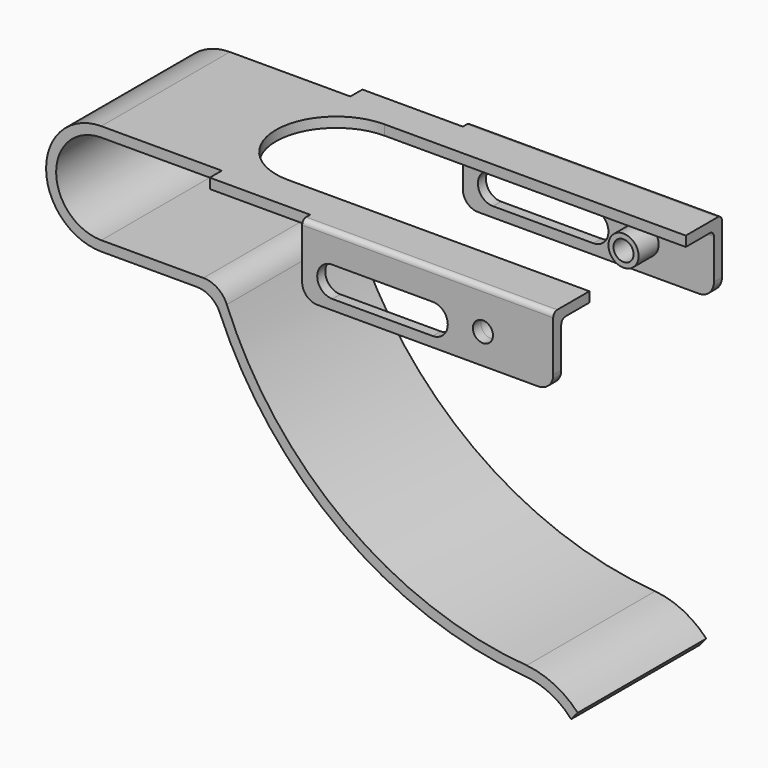
from build123d import *

# Parameters (mm, degrees)
F1_DEPTH  = 16
F2_W      = 70
F2_H      = 3
F3_DEPTH  = 2
F4_W      = 50
F4_H      = 14
F5_DEPTH  = 2
F6_R      = 1
F9_DEPTH  = 2
F11_DEPTH = 42.001
F13_D     = 4
F14_R     = 3
F14_R_2   = 2
F15_DEPTH = 5
F16_R     = 3


# Not quite as in the source:
# - a pattern or mirror of a feature is missing from the dataset's text; its kind, count and spacing are read off the source's solid


with BuildPart() as f1:
    # F0 (on Front) → F1 (new body)
    with BuildSketch(Plane.XZ):
        with BuildLine():
            ThreePointArc((0, -9), (-9, 0), (0, 9))
            Line((0, 9), (94, 9))
            Line((94, 9), (94, 11))
            Line((94, 11), (0, 11))
            ThreePointArc((0, 11), (-11, 0), (0, -11))
            Line((0, -11), (19, -11))
            ThreePointArc((19, -11), (21.7681124643, -11.8361612201), (23.6103896104, -14.064978646))
            ThreePointArc((23.6103896104, -14.064978646), (47.704208574, -44.4678662727), (84.0759449666, -57.9565459739))
            ThreePointArc((84.0759449666, -57.9565459739), (89.2804195373, -59.3196982134), (93.5865207758, -62.5449473062))
            Line((93.5865207758, -62.5449473062), (94.8828854905, -61))
            ThreePointArc((94.8828854905, -61), (90.2510294077, -57.5678191663), (84.7034264019, -56))
            ThreePointArc((84.7034264019, -56), (48.5673164119, -42.6217020739), (24.9861322889, -12.1467114099))
            ThreePointArc((24.9861322889, -12.1467114099), (23.1470623984, -9.8607704249), (20.3422845953, -9))
            Line((20.3422845953, -9), (0, -9))
        make_face()
    extrude(amount=F1_DEPTH)

    # F2 (on face) → F3 (join)
    with BuildSketch(Plane.XY.offset(11)):
        with Locations((59, -17.5)):
            Rectangle(F2_W, F2_H)
    extrude(amount=-F3_DEPTH)

    # F4 (on face) → F5 (join)
    with BuildSketch(Plane.XZ.offset(19)):
        with Locations((69, 4)):
            Rectangle(F4_W, F4_H)
    extrude(amount=F5_DEPTH)

    # F6
    f6_edges = [f1.edges().sort_by_distance(p)[0] for p in [
        (69, -21, 11),
        (69, -19, 9),
    ]]
    fillet(f6_edges, radius=F6_R)

    # F7: F1 across plane


with BuildPart() as f1_1:
    add(f1.part)
    add(f1.part.mirror(Plane.XZ))

    # F8 (on face) → F9 (cut)
    with BuildSketch(Plane.XY.offset(11)):
        with BuildLine():
            Line((94, 12), (34, 12))
            ThreePointArc((34, 12), (22, 0), (34, -12))
            Line((34, -12), (94, -12))
            Line((94, -12), (94, 12))
        make_face()
    extrude(amount=-F9_DEPTH, mode=Mode.SUBTRACT)

    # F10 (on face) → F11 (cut, through all)
    with BuildSketch(Plane.XZ.offset(21)):
        with BuildLine():
            ThreePointArc((50, 5), (47, 2), (50, -1))
            Line((50, -1), (70, -1))
            ThreePointArc((70, -1), (73, 2), (70, 5))
            Line((70, 5), (50, 5))
        make_face()
    extrude(amount=-F11_DEPTH, mode=Mode.SUBTRACT)

    # F13 (through all)
    with Locations(Plane.XZ.offset(21)):
        with Locations((80, 3)):
            Hole(F13_D / 2)

    # F14 (on face) → F15 (join)
    with BuildSketch(Plane(origin=(0, -19, 0), x_dir=(-1, 0, 0), z_dir=(0, 1, 0))):
        with Locations((-80, 3)):
            Circle(F14_R)
        with Locations((-80, 3)):
            Circle(F14_R_2, mode=Mode.SUBTRACT)
    f15 = extrude(amount=F15_DEPTH)

    # F15_copies: F15 across plane
    add(f15.mirror(Plane.ZX))

    # F16
    f16_edges = [f1_1.edges().sort_by_distance(p)[0] for p in [
        (94, 20, -3),
        (44, 20, -3),
        (44, -20, -3),
        (94, -20, -3),
    ]]
    fillet(f16_edges, radius=F16_R)


solid = f1_1.part
